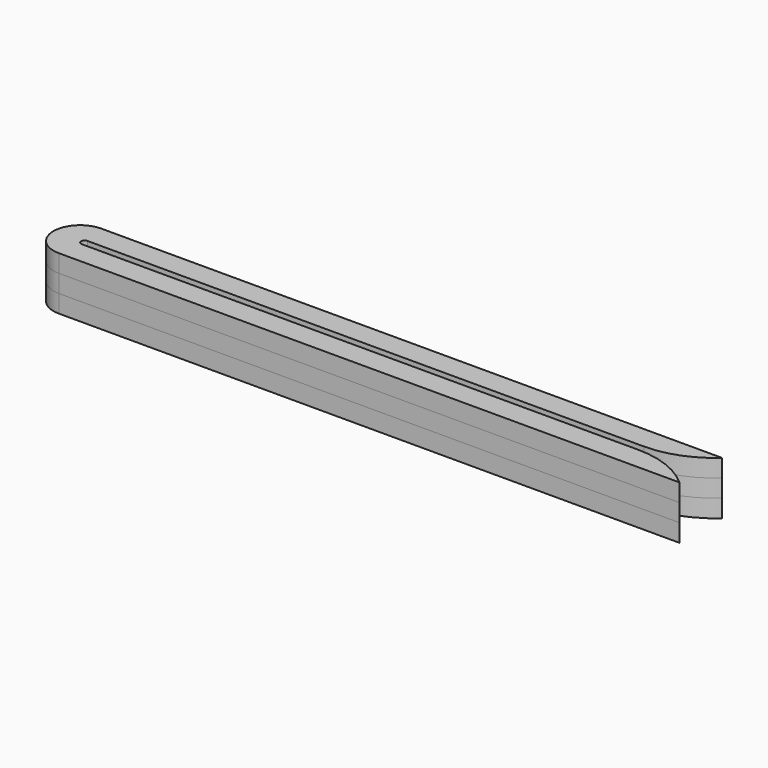
from build123d import *

# Parameters (mm, degrees)
F1_DEPTH      = 1
F2_DEPTH      = 1
F3_DEPTH      = 1
F4_T1_DEPTH   = 17.8151717208
F4_2_T1_DEPTH = 17.8151717208
F4_3_T1_DEPTH = 17.8151717208


# Not quite as in the source:
# - a fillet or chamfer that OpenCascade refuses, or shapes differently, is made with other operations: its cross-section is extruded or revolved along the edge and cut away or added


with BuildPart() as f1:
    # F0 (on Top) → F1 (new body)
    with BuildSketch(Plane.XY):
        with BuildLine():
            Line((35, 1.5), (0, 1.5))
            ThreePointArc((0, 1.5), (-1.5, 0), (0, -1.5))
            Line((0, -1.5), (35, -1.5))
            Line((35, -1.5), (35, -0.2))
            Line((35, -0.2), (0.254249986, -0.2))
            ThreePointArc((0.254249986, -0.2), (0.054249986, 0), (0.254249986, 0.2))
            Line((0.254249986, 0.2), (35, 0.2))
            Line((35, 0.2), (35, 1.5))
        make_face()
    extrude(amount=F1_DEPTH)


with BuildPart() as f2:
    # F2 (new): a face of the model
    f2_faces = [f1.part.faces().sort_by_distance(p)[0] for p in [
        (34.6337691985, 0.85, 1),
    ]]
    extrude(f2_faces, amount=F2_DEPTH)


with BuildPart() as f3:
    # F3 (new): a face of the model
    f3_faces = [f2.part.faces().sort_by_distance(p)[0] for p in [
        (34.6337691985, 0.85, 2),
    ]]
    extrude(f3_faces, amount=F3_DEPTH)

    # F4#3: fillet of radius 5 on 2 edges, made by hand

    # F4_3_s2 → F4_3_t1 (cut)
    with BuildSketch(Plane.XY.offset(-6.4075858604)):
        with BuildLine():
            ThreePointArc((35, -1.5), (33.4397412936, -0.5363104735), (31.6369656558, -0.2))
            Line((31.6369656558, -0.2), (35, -0.2))
            Line((35, -0.2), (35, -1.5))
        make_face()
        with BuildLine():
            ThreePointArc((35, 1.5), (33.4397412936, 0.5363104735), (31.6369656558, 0.2))
            Line((31.6369656558, 0.2), (35, 0.2))
            Line((35, 0.2), (35, 1.5))
        make_face()
    extrude(amount=F4_3_T1_DEPTH, mode=Mode.SUBTRACT)


with BuildPart() as f1_1:
    add(f1.part)

    # F4: fillet of radius 5 on 2 edges, made by hand

    # F4_s2 → F4_t1 (cut)
    with BuildSketch(Plane.XY.offset(-8.4075858604)):
        with BuildLine():
            ThreePointArc((35, 1.5), (33.4397412936, 0.5363104735), (31.6369656558, 0.2))
            Line((31.6369656558, 0.2), (35, 0.2))
            Line((35, 0.2), (35, 1.5))
        make_face()
        with BuildLine():
            ThreePointArc((35, -1.5), (33.4397412936, -0.5363104735), (31.6369656558, -0.2))
            Line((31.6369656558, -0.2), (35, -0.2))
            Line((35, -0.2), (35, -1.5))
        make_face()
    extrude(amount=F4_T1_DEPTH, mode=Mode.SUBTRACT)


with BuildPart() as f2_1:
    add(f2.part)

    # F4#2: fillet of radius 5 on 2 edges, made by hand

    # F4_2_s2 → F4_2_t1 (cut)
    with BuildSketch(Plane.XY.offset(-7.4075858604)):
        with BuildLine():
            ThreePointArc((35, 1.5), (33.4397412936, 0.5363104735), (31.6369656558, 0.2))
            Line((31.6369656558, 0.2), (35, 0.2))
            Line((35, 0.2), (35, 1.5))
        make_face()
        with BuildLine():
            ThreePointArc((35, -1.5), (33.4397412936, -0.5363104735), (31.6369656558, -0.2))
            Line((31.6369656558, -0.2), (35, -0.2))
            Line((35, -0.2), (35, -1.5))
        make_face()
    extrude(amount=F4_2_T1_DEPTH, mode=Mode.SUBTRACT)


solid = Compound([f3.part, f1_1.part, f2_1.part])
